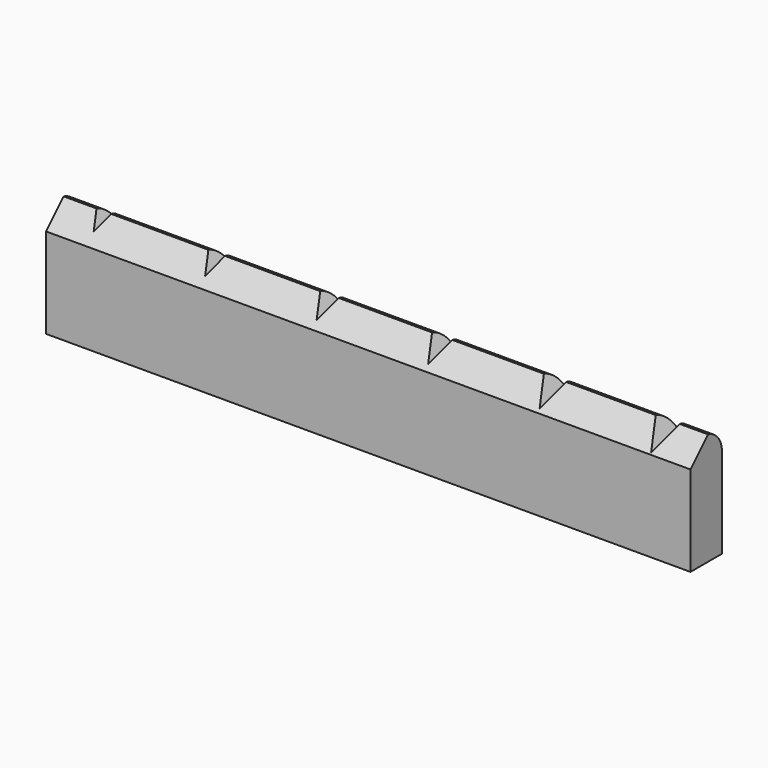
from build123d import *

# Parameters (mm, degrees)
F0_W        = 50.8
F0_H        = 3.0988
F1_DEPTH    = 8.89
F3_R        = 1.778
F4_T1_DEPTH = 59.9449047052
F5_DEPTH    = 25.4


# Not quite as in the source:
# - a fillet or chamfer that OpenCascade refuses, or shapes differently, is made with other operations: its cross-section is extruded or revolved along the edge and cut away or added


with BuildPart() as f1:
    # F0 (on Top) → F1 (new body)
    with BuildSketch(Plane.XY):
        with Locations((0, 1.5494)):
            Rectangle(F0_W, F0_H)
    extrude(amount=F1_DEPTH)

    # F3
    f3_edges = [f1.edges().sort_by_distance(p)[0] for p in [
        (0, 3.0988, 8.89),
    ]]
    fillet(f3_edges, radius=F3_R)

    # F4: chamfer of 1.778 on 1 edges, made by hand

    # F4_s2 → F4_t1 (cut)
    with BuildSketch(Plane.YZ.offset(-29.9724523526)):
        Polygon((1.778, 8.89), (0, 7.112), (0, 8.89), align=None)
    extrude(amount=F4_T1_DEPTH, mode=Mode.SUBTRACT)

    # F2 (on face) → F5 (cut)
    with BuildSketch(Plane.XZ):
        Polygon((-22.225, 7.8332954744), (-21.6149113577, 8.89), (-22.8350886423, 8.89), align=None)
        Polygon((-12.6515878735, 8.89), (-14.0184121265, 8.89), (-13.335, 7.7062954744), align=None)
        Polygon((14.2383825791, 8.89), (12.4316174209, 8.89), (13.335, 7.3252954744), align=None)
        Polygon((22.225, 7.1982954744), (23.2017060633, 8.89), (21.2482939367, 8.89), align=None)
        Polygon((-3.6882643893, 8.89), (-5.2017356107, 8.89), (-4.445, 7.5792954744), align=None)
        Polygon((5.2750590949, 8.89), (3.6149409051, 8.89), (4.445, 7.4522954744), align=None)
    extrude(amount=-F5_DEPTH, mode=Mode.SUBTRACT)


solid = f1.part
